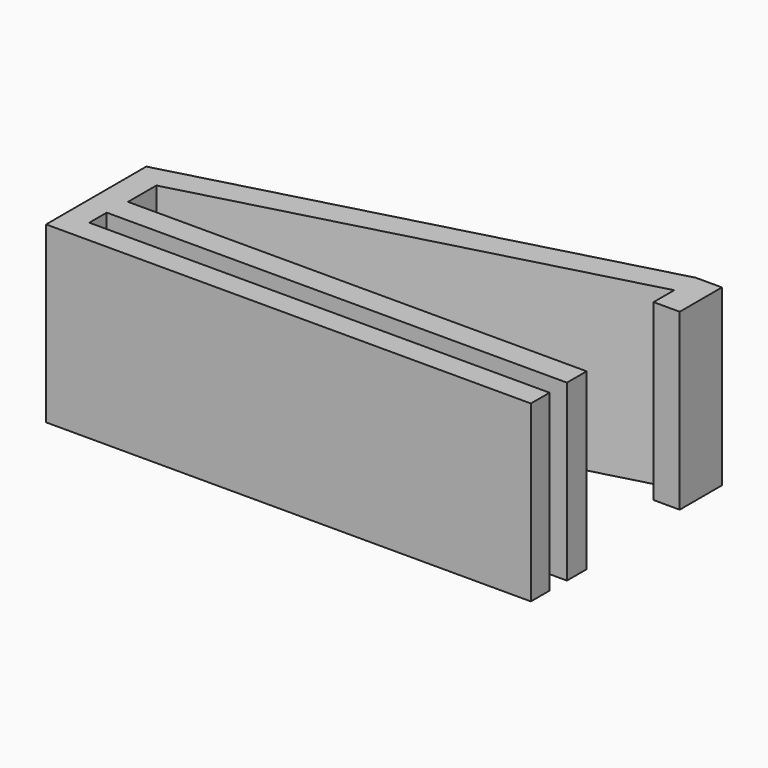
from build123d import *

# Parameters (mm, degrees)
F0_W          = 55.6310900272
F0_H          = 20
F1_DEPTH      = 8
F2_W          = 2.5
F2_H          = 40
F3_DEPTH      = 27.8165450136
F3_DEPTH_BACK = 25
F5_DEPTH      = 10


# Not quite as in the source:
# - a feature names something its author has since deleted; it is built from what else it names


with BuildPart() as f1:
    # F0 (on Front) → F1 (new body)
    with BuildSketch(Plane.XZ):
        Rectangle(F0_W, F0_H)
    extrude(amount=-F1_DEPTH)

    # F2 (on Right) → F3 (cut, two sides)
    with BuildSketch(Plane.YZ) as f3_sk:
        with Locations((3.9288233686, 0)):
            Rectangle(F2_W, F2_H)
    extrude(amount=F3_DEPTH, mode=Mode.SUBTRACT)
    extrude(f3_sk.sketch, amount=-F3_DEPTH_BACK, mode=Mode.SUBTRACT)

    # F4 (on Top) → F5 (join, symmetric)
    with BuildSketch(Plane.XY):
        Polygon((24.1118337571, 28.2883709489), (-27.8155450136, 14.3744717422), (-27.8155450136, 8), (-24.8155450136, 8), (-24.8155450136, 12.0724907783), (24.1118337571, 25.1825424077), align=None)
        Polygon((27.1118309825, 28.2842907635), (24.1118337571, 28.2883709489), (24.1118337571, 25.1825424077), (24.1118337571, 22.2315117717), (27.1118309825, 22.2315117717), align=None)
    extrude(amount=F5_DEPTH, both=True)


solid = f1.part
